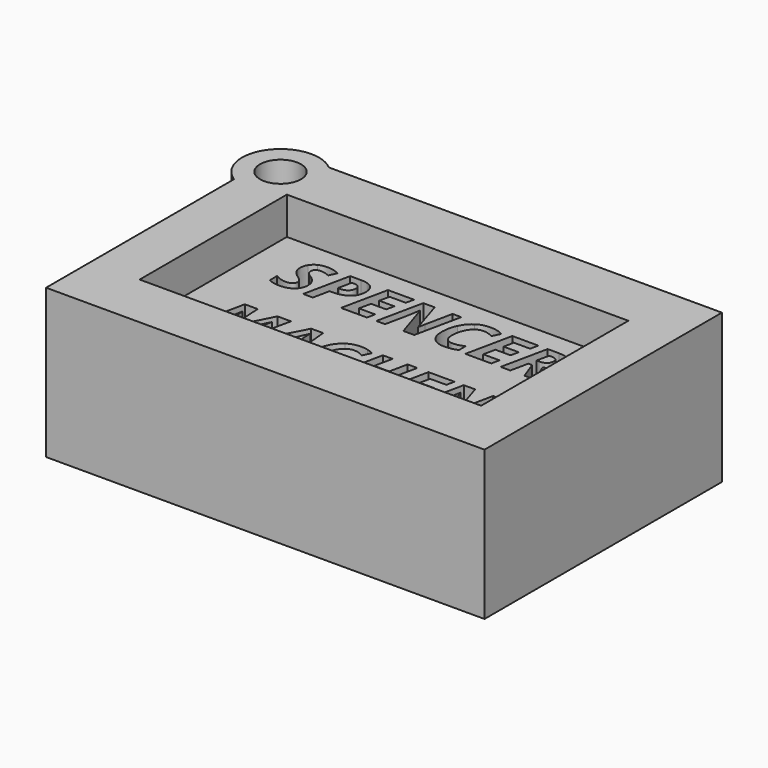
from build123d import *

# Parameters (mm, degrees)
F0_W         = 58.1890940666
F0_H         = 31.3483476639
F1_DEPTH     = 6.35
F2_DEPTH     = 25.4
F3_DEPTH     = 12.7
F4_DEPTH     = 12.7
F0_TEXT_SIZE = 11.0982710289
F5_DEPTH     = 12.7
F6_DEPTH     = 19.05


# Not quite as in the source:
# - Text() gives the source's letters only with a copy of the font that has no kerning and outlines rounded to 1/6400 em; it was checked with that copy


with BuildPart() as f1:
    # F0 (on Top) → F1 (new body)
    with BuildSketch(Plane.XY):
        with BuildLine():
            Line((-37.3486888398, -25.2818514363), (37.3486888398, -25.2818514363))
            Line((37.3486888398, -25.2818514363), (37.3486888398, 25.2818514363))
            Line((37.3486888398, 25.2818514363), (-29.6175755934, 25.2818514363))
            ThreePointArc((-29.6175755934, 25.2818514363), (-27.9167987863, 23.0401985803), (-27.3127590842, 20.2919654548))
            ThreePointArc((-27.3127590842, 20.2919654548), (-30.6939014972, 14.5572193058), (-37.3486888398, 14.7395454853))
            Line((-37.3486888398, 14.7395454853), (-37.3486888398, -25.2818514363))
        make_face()
        Rectangle(F0_W, F0_H, mode=Mode.SUBTRACT)
        Rectangle(F0_W, F0_H)
        with BuildLine():
            Line((-18.7833381513, -8.8915199012), (-18.7607947882, -8.8915199012))
            Line((-18.7607947882, -8.8915199012), (-15.7746662395, -2.9678177396))
            Line((-15.7746662395, -2.9678177396), (-13.4821796301, -2.9678177396))
            Line((-13.4821796301, -2.9678177396), (-15.1573249136, -10.8909427913))
            Line((-15.1573249136, -10.8909427913), (-16.6746666558, -10.8909427913))
            Line((-16.6746666558, -10.8909427913), (-15.8891171595, -7.1400740045))
            add(Edge.make_bspline(
                [(-15.8891171595, -7.1400740045), (-15.6012557547, -5.8030791665), (-15.3203307693, -4.7504775236)],
                knots=[0, 0, 0, 1, 1, 1], degree=2))
            Line((-15.3203307693, -4.7504775236), (-15.346342342, -4.7504775236))
            Line((-15.346342342, -4.7504775236), (-18.4313148671, -10.8909427913))
            Line((-18.4313148671, -10.8909427913), (-19.9538589239, -10.8909427913))
            Line((-19.9538589239, -10.8909427913), (-20.283338845, -4.7504775236))
            Line((-20.283338845, -4.7504775236), (-20.305882208, -4.7504775236))
            add(Edge.make_bspline(
                [(-20.305882208, -4.7504775236), (-20.3648417729, -5.2273563569), (-20.5113736326, -6.002501224)],
                knots=[0, 0, 0, 1, 1, 1], degree=2))
            add(Edge.make_bspline(
                [(-20.5113736326, -6.002501224), (-20.6579054922, -6.7776460912), (-21.5249579164, -10.8909427913)],
                knots=[0, 0, 0, 1, 1, 1], degree=2))
            Line((-21.5249579164, -10.8909427913), (-23.014553981, -10.8909427913))
            Line((-23.014553981, -10.8909427913), (-21.3411428025, -2.9678177396))
            Line((-21.3411428025, -2.9678177396), (-19.1509683791, -2.9678177396))
            Line((-19.1509683791, -2.9678177396), (-18.7833381513, -8.8915199012))
        make_face(mode=Mode.SUBTRACT)
        Polygon((-8.8451832659, -10.8909427913), (-8.9752411295, -9.0042367164), (-11.5382480952, -9.0042367164), (-12.4694623988, -10.8909427913), (-14.203567247, -10.8909427913), (-10.0538543451, -2.9348697475), (-8.0318880921, -2.9348697475), (-7.2359339667, -10.8909427913), align=None, mode=Mode.SUBTRACT)
        with BuildLine():
            add(Edge.make_bspline(
                [(-0.9211911618, -4.3446969891), (-1.2948907566, -4.242384803), (-1.6642550893, -4.242384803)],
                knots=[0, 0, 0, 1, 1, 1], degree=2))
            add(Edge.make_bspline(
                [(-1.6642550893, -4.242384803), (-2.3787062867, -4.242384803), (-2.9509608867, -4.6811133297)],
                knots=[0, 0, 0, 1, 1, 1], degree=2))
            add(Edge.make_bspline(
                [(-2.9509608867, -4.6811133297), (-3.5232154866, -5.1198418563), (-3.8700364562, -5.9730214416)],
                knots=[0, 0, 0, 1, 1, 1], degree=2))
            add(Edge.make_bspline(
                [(-3.8700364562, -5.9730214416), (-4.2168574259, -6.8262010269), (-4.2168574259, -7.8077043711)],
                knots=[0, 0, 0, 1, 1, 1], degree=2))
            add(Edge.make_bspline(
                [(-4.2168574259, -7.8077043711), (-4.2168574259, -8.7129071019), (-3.8457589884, -9.1516356285)],
                knots=[0, 0, 0, 1, 1, 1], degree=2))
            add(Edge.make_bspline(
                [(-3.8457589884, -9.1516356285), (-3.4746605508, -9.5903641551), (-2.661365377, -9.5903641551)],
                knots=[0, 0, 0, 1, 1, 1], degree=2))
            add(Edge.make_bspline(
                [(-2.661365377, -9.5903641551), (-1.8706135662, -9.5903641551), (-0.8301506572, -9.1724448866)],
                knots=[0, 0, 0, 1, 1, 1], degree=2))
            Line((-0.8301506572, -9.1724448866), (-0.8301506572, -10.5822721283))
            add(Edge.make_bspline(
                [(-0.8301506572, -10.5822721283), (-1.907029768, -11.0001913967), (-2.9977817176, -11.0001913967)],
                knots=[0, 0, 0, 1, 1, 1], degree=2))
            add(Edge.make_bspline(
                [(-2.9977817176, -11.0001913967), (-4.3729268622, -11.0001913967), (-5.1376671003, -10.1894973801)],
                knots=[0, 0, 0, 1, 1, 1], degree=2))
            add(Edge.make_bspline(
                [(-5.1376671003, -10.1894973801), (-5.9024073384, -9.3788033636), (-5.9024073384, -7.8944096135)],
                knots=[0, 0, 0, 1, 1, 1], degree=2))
            add(Edge.make_bspline(
                [(-5.9024073384, -7.8944096135), (-5.9024073384, -6.4741777428), (-5.3388232627, -5.2793795023)],
                knots=[0, 0, 0, 1, 1, 1], degree=2))
            add(Edge.make_bspline(
                [(-5.3388232627, -5.2793795023), (-4.775239187, -4.0845812618), (-3.8318861496, -3.4637717262)],
                knots=[0, 0, 0, 1, 1, 1], degree=2))
            add(Edge.make_bspline(
                [(-3.8318861496, -3.4637717262), (-2.8885331121, -2.8429621905), (-1.6642550893, -2.8429621905)],
                knots=[0, 0, 0, 1, 1, 1], degree=2))
            add(Edge.make_bspline(
                [(-1.6642550893, -2.8429621905), (-0.9862200936, -2.8429621905), (-0.4607863246, -2.9652165823)],
                knots=[0, 0, 0, 1, 1, 1], degree=2))
            add(Edge.make_bspline(
                [(-0.4607863246, -2.9652165823), (0.0646474445, -3.0874709741), (0.6663818268, -3.4117485807)],
                knots=[0, 0, 0, 1, 1, 1], degree=2))
            Line((0.6663818268, -3.4117485807), (0.0264971378, -4.7678185721))
            add(Edge.make_bspline(
                [(0.0264971378, -4.7678185721), (-0.547491567, -4.4470091751), (-0.9211911618, -4.3446969891)],
                knots=[0, 0, 0, 1, 1, 1], degree=2))
        make_face(mode=Mode.SUBTRACT)
        Polygon((8.0484661658, -2.9678177396), (6.3733208824, -10.8909427913), (4.7155166475, -10.8909427913), (5.4403724741, -7.4712880305), (2.8895042423, -7.4712880305), (2.1629143109, -10.8909427913), (0.5103123905, -10.8909427913), (2.183723569, -2.9678177396), (3.8432619088, -2.9678177396), (3.1860361713, -6.0735995228), (5.738638508, -6.0735995228), (6.3941301406, -2.9678177396), align=None, mode=Mode.SUBTRACT)
        Polygon((13.0010696125, -9.5036589127), (12.7080058931, -10.8909427913), (8.2808362155, -10.8909427913), (9.9542473941, -2.9678177396), (14.3883534911, -2.9678177396), (14.0952897717, -4.3446969891), (11.3207220145, -4.3446969891), (10.9565599964, -6.0840041519), (13.5421103251, -6.0840041519), (13.2438442912, -7.4608834014), (10.6600280673, -7.4608834014), (10.2265018553, -9.5036589127), align=None, mode=Mode.SUBTRACT)
        with BuildLine():
            Line((22.4415364064, -2.9678177396), (20.766391123, -10.8909427913))
            Line((20.766391123, -10.8909427913), (18.9126330402, -10.8909427913))
            Line((18.9126330402, -10.8909427913), (16.9843084489, -4.8978764357))
            Line((16.9843084489, -4.8978764357), (16.9513604568, -4.8978764357))
            Line((16.9513604568, -4.8978764357), (16.9288170938, -5.0712869205))
            add(Edge.make_bspline(
                [(16.9288170938, -5.0712869205), (16.755406609, -6.2418076931), (16.571591495, -7.1626173675)],
                knots=[0, 0, 0, 1, 1, 1], degree=2))
            Line((16.571591495, -7.1626173675), (15.7860419988, -10.8909427913))
            Line((15.7860419988, -10.8909427913), (14.2964459341, -10.8909427913))
            Line((14.2964459341, -10.8909427913), (15.9698571127, -2.9678177396))
            Line((15.9698571127, -2.9678177396), (17.9051181234, -2.9678177396))
            Line((17.9051181234, -2.9678177396), (19.7467374722, -8.8048146588))
            Line((19.7467374722, -8.8048146588), (19.7692808352, -8.8048146588))
            add(Edge.make_bspline(
                [(19.7692808352, -8.8048146588), (19.8334427146, -8.3920977049), (19.9799745743, -7.6282245193)],
                knots=[0, 0, 0, 1, 1, 1], degree=2))
            add(Edge.make_bspline(
                [(19.9799745743, -7.6282245193), (20.126506434, -6.8643513336), (20.9554085514, -2.9678177396)],
                knots=[0, 0, 0, 1, 1, 1], degree=2))
            Line((20.9554085514, -2.9678177396), (22.4415364064, -2.9678177396))
        make_face(mode=Mode.SUBTRACT)
        with BuildLine():
            add(Edge.make_bspline(
                [(-18.5015461134, 7.7654242187), (-18.1764014544, 7.242591607), (-18.1764014544, 6.5437473531)],
                knots=[0, 0, 0, 1, 1, 1], degree=2))
            add(Edge.make_bspline(
                [(-18.1764014544, 6.5437473531), (-18.1764014544, 5.4113768872), (-18.9784249467, 4.7524170449)],
                knots=[0, 0, 0, 1, 1, 1], degree=2))
            add(Edge.make_bspline(
                [(-18.9784249467, 4.7524170449), (-19.780448439, 4.0934572025), (-21.1503912692, 4.0934572025)],
                knots=[0, 0, 0, 1, 1, 1], degree=2))
            add(Edge.make_bspline(
                [(-21.1503912692, 4.0934572025), (-22.3486577193, 4.0934572025), (-23.0804499653, 4.5824747698)],
                knots=[0, 0, 0, 1, 1, 1], degree=2))
            Line((-23.0804499653, 4.5824747698), (-23.0804499653, 6.0668685199))
            add(Edge.make_bspline(
                [(-23.0804499653, 6.0668685199), (-22.0347847418, 5.482475186), (-21.1399866401, 5.482475186)],
                knots=[0, 0, 0, 1, 1, 1], degree=2))
            add(Edge.make_bspline(
                [(-21.1399866401, 5.482475186), (-20.5330499432, 5.482475186), (-20.1914312881, 5.7122440784)],
                knots=[0, 0, 0, 1, 1, 1], degree=2))
            add(Edge.make_bspline(
                [(-20.1914312881, 5.7122440784), (-19.849812633, 5.9420129708), (-19.849812633, 6.3425911907)],
                knots=[0, 0, 0, 1, 1, 1], degree=2))
            add(Edge.make_bspline(
                [(-19.849812633, 6.3425911907), (-19.849812633, 6.5766953453), (-19.923512089, 6.7527069873)],
                knots=[0, 0, 0, 1, 1, 1], degree=2))
            add(Edge.make_bspline(
                [(-19.923512089, 6.7527069873), (-19.9972115451, 6.9287186294), (-20.1324717232, 7.0804528037)],
                knots=[0, 0, 0, 1, 1, 1], degree=2))
            add(Edge.make_bspline(
                [(-20.1324717232, 7.0804528037), (-20.2677319014, 7.2321869779), (-20.8035702995, 7.6327651978)],
                knots=[0, 0, 0, 1, 1, 1], degree=2))
            add(Edge.make_bspline(
                [(-20.8035702995, 7.6327651978), (-21.5527035939, 8.1703377008), (-21.8561719424, 8.6957714698)],
                knots=[0, 0, 0, 1, 1, 1], degree=2))
            add(Edge.make_bspline(
                [(-21.8561719424, 8.6957714698), (-22.1596402908, 9.2212052388), (-22.1596402908, 9.8281419357)],
                knots=[0, 0, 0, 1, 1, 1], degree=2))
            add(Edge.make_bspline(
                [(-22.1596402908, 9.8281419357), (-22.1596402908, 10.5269861896), (-21.8232239503, 11.0766974265)],
                knots=[0, 0, 0, 1, 1, 1], degree=2))
            add(Edge.make_bspline(
                [(-21.8232239503, 11.0766974265), (-21.4868076097, 11.6264086634), (-20.865998074, 11.9324781691)],
                knots=[0, 0, 0, 1, 1, 1], degree=2))
            add(Edge.make_bspline(
                [(-20.865998074, 11.9324781691), (-20.2451885384, 12.2385476748), (-19.4388297839, 12.2385476748)],
                knots=[0, 0, 0, 1, 1, 1], degree=2))
            add(Edge.make_bspline(
                [(-19.4388297839, 12.2385476748), (-18.2631066968, 12.2385476748), (-17.2868056672, 11.7027092767)],
                knots=[0, 0, 0, 1, 1, 1], degree=2))
            Line((-17.2868056672, 11.7027092767), (-17.8781354205, 10.4402809472))
            add(Edge.make_bspline(
                [(-17.8781354205, 10.4402809472), (-18.7226444816, 10.8408591671), (-19.4388297839, 10.8408591671)],
                knots=[0, 0, 0, 1, 1, 1], degree=2))
            add(Edge.make_bspline(
                [(-19.4388297839, 10.8408591671), (-19.8879629396, 10.8408591671), (-20.174957292, 10.5972174359)],
                knots=[0, 0, 0, 1, 1, 1], degree=2))
            add(Edge.make_bspline(
                [(-20.174957292, 10.5972174359), (-20.4619516444, 10.3535757048), (-20.4619516444, 9.9529974848)],
                knots=[0, 0, 0, 1, 1, 1], degree=2))
            add(Edge.make_bspline(
                [(-20.4619516444, 9.9529974848), (-20.4619516444, 9.6217834588), (-20.283338845, 9.3755405703)],
                knots=[0, 0, 0, 1, 1, 1], degree=2))
            add(Edge.make_bspline(
                [(-20.283338845, 9.3755405703), (-20.1047260457, 9.1292976819), (-19.4821824051, 8.7217830425)],
                knots=[0, 0, 0, 1, 1, 1], degree=2))
            add(Edge.make_bspline(
                [(-19.4821824051, 8.7217830425), (-18.8266907725, 8.2882568305), (-18.5015461134, 7.7654242187)],
                knots=[0, 0, 0, 1, 1, 1], degree=2))
        make_face(mode=Mode.SUBTRACT)
        with BuildLine():
            add(Edge.make_bspline(
                [(-11.6448955434, 11.5483739452), (-10.9729299147, 10.9709170307), (-10.9729299147, 9.8177373066)],
                knots=[0, 0, 0, 1, 1, 1], degree=2))
            add(Edge.make_bspline(
                [(-10.9729299147, 9.8177373066), (-10.9729299147, 8.5102222511), (-11.8920054843, 7.7654242187)],
                knots=[0, 0, 0, 1, 1, 1], degree=2))
            add(Edge.make_bspline(
                [(-11.8920054843, 7.7654242187), (-12.8110810539, 7.0206261864), (-14.4255326676, 7.0206261864)],
                knots=[0, 0, 0, 1, 1, 1], degree=2))
            Line((-14.4255326676, 7.0206261864), (-14.8920068718, 7.0206261864))
            Line((-14.8920068718, 7.0206261864), (-15.4816025202, 4.202705808))
            Line((-15.4816025202, 4.202705808), (-17.1342044406, 4.202705808))
            Line((-17.1342044406, 4.202705808), (-15.460793262, 12.1258308597))
            Line((-15.460793262, 12.1258308597), (-13.6278444374, 12.1258308597))
            add(Edge.make_bspline(
                [(-13.6278444374, 12.1258308597), (-12.3168611721, 12.1258308597), (-11.6448955434, 11.5483739452)],
                knots=[0, 0, 0, 1, 1, 1], degree=2))
        make_face(mode=Mode.SUBTRACT)
        Polygon((-5.975239742, 5.5899896866), (-6.2683034614, 4.202705808), (-10.695473139, 4.202705808), (-9.0220619604, 12.1258308597), (-4.5879558634, 12.1258308597), (-4.8810195828, 10.7489516102), (-7.65558734, 10.7489516102), (-8.0197493581, 9.0096444474), (-5.4341990294, 9.0096444474), (-5.7324650633, 7.6327651978), (-8.3162812872, 7.6327651978), (-8.7498074992, 5.5899896866), align=None, mode=Mode.SUBTRACT)
        with BuildLine():
            Line((3.4652270519, 12.1258308597), (1.7900817685, 4.202705808))
            Line((1.7900817685, 4.202705808), (-0.0636763143, 4.202705808))
            Line((-0.0636763143, 4.202705808), (-1.9920009056, 10.1957721636))
            Line((-1.9920009056, 10.1957721636), (-2.0249488977, 10.1957721636))
            Line((-2.0249488977, 10.1957721636), (-2.0474922607, 10.0223616787))
            add(Edge.make_bspline(
                [(-2.0474922607, 10.0223616787), (-2.2209027455, 8.8518409062), (-2.4047178595, 7.9310312317)],
                knots=[0, 0, 0, 1, 1, 1], degree=2))
            Line((-2.4047178595, 7.9310312317), (-3.1902673557, 4.202705808))
            Line((-3.1902673557, 4.202705808), (-4.6798634204, 4.202705808))
            Line((-4.6798634204, 4.202705808), (-3.0064522418, 12.1258308597))
            Line((-3.0064522418, 12.1258308597), (-1.0711912312, 12.1258308597))
            Line((-1.0711912312, 12.1258308597), (0.7704281177, 6.2888339404))
            Line((0.7704281177, 6.2888339404), (0.7929714807, 6.2888339404))
            add(Edge.make_bspline(
                [(0.7929714807, 6.2888339404), (0.8571333601, 6.7015508943), (1.0036652198, 7.46542408)],
                knots=[0, 0, 0, 1, 1, 1], degree=2))
            add(Edge.make_bspline(
                [(1.0036652198, 7.46542408), (1.1501970795, 8.2292972656), (1.9790991969, 12.1258308597)],
                knots=[0, 0, 0, 1, 1, 1], degree=2))
            Line((1.9790991969, 12.1258308597), (3.4652270519, 12.1258308597))
        make_face(mode=Mode.SUBTRACT)
        with BuildLine():
            add(Edge.make_bspline(
                [(9.0568481351, 10.7489516102), (8.6831485403, 10.8512637962), (8.3137842076, 10.8512637962)],
                knots=[0, 0, 0, 1, 1, 1], degree=2))
            add(Edge.make_bspline(
                [(8.3137842076, 10.8512637962), (7.5993330101, 10.8512637962), (7.0270784102, 10.4125352696)],
                knots=[0, 0, 0, 1, 1, 1], degree=2))
            add(Edge.make_bspline(
                [(7.0270784102, 10.4125352696), (6.4548238103, 9.973806743), (6.1080028406, 9.1206271576)],
                knots=[0, 0, 0, 1, 1, 1], degree=2))
            add(Edge.make_bspline(
                [(6.1080028406, 9.1206271576), (5.761181871, 8.2674475723), (5.761181871, 7.2859442282)],
                knots=[0, 0, 0, 1, 1, 1], degree=2))
            add(Edge.make_bspline(
                [(5.761181871, 7.2859442282), (5.761181871, 6.3807414974), (6.1322803085, 5.9420129708)],
                knots=[0, 0, 0, 1, 1, 1], degree=2))
            add(Edge.make_bspline(
                [(6.1322803085, 5.9420129708), (6.503378746, 5.5032844442), (7.3166739199, 5.5032844442)],
                knots=[0, 0, 0, 1, 1, 1], degree=2))
            add(Edge.make_bspline(
                [(7.3166739199, 5.5032844442), (8.1074257307, 5.5032844442), (9.1478886396, 5.9212037126)],
                knots=[0, 0, 0, 1, 1, 1], degree=2))
            Line((9.1478886396, 5.9212037126), (9.1478886396, 4.511376471))
            add(Edge.make_bspline(
                [(9.1478886396, 4.511376471), (8.0710095289, 4.0934572025), (6.9802575793, 4.0934572025)],
                knots=[0, 0, 0, 1, 1, 1], degree=2))
            add(Edge.make_bspline(
                [(6.9802575793, 4.0934572025), (5.6051124346, 4.0934572025), (4.8403721966, 4.9041512191)],
                knots=[0, 0, 0, 1, 1, 1], degree=2))
            add(Edge.make_bspline(
                [(4.8403721966, 4.9041512191), (4.0756319585, 5.7148452357), (4.0756319585, 7.1992389858)],
                knots=[0, 0, 0, 1, 1, 1], degree=2))
            add(Edge.make_bspline(
                [(4.0756319585, 7.1992389858), (4.0756319585, 8.6194708565), (4.6392160342, 9.814269097)],
                knots=[0, 0, 0, 1, 1, 1], degree=2))
            add(Edge.make_bspline(
                [(4.6392160342, 9.814269097), (5.2028001099, 11.0090673374), (6.1461531473, 11.6298768731)],
                knots=[0, 0, 0, 1, 1, 1], degree=2))
            add(Edge.make_bspline(
                [(6.1461531473, 11.6298768731), (7.0895061848, 12.2506864088), (8.3137842076, 12.2506864088)],
                knots=[0, 0, 0, 1, 1, 1], degree=2))
            add(Edge.make_bspline(
                [(8.3137842076, 12.2506864088), (8.9918192033, 12.2506864088), (9.5172529723, 12.128432017)],
                knots=[0, 0, 0, 1, 1, 1], degree=2))
            add(Edge.make_bspline(
                [(9.5172529723, 12.128432017), (10.0426867413, 12.0061776252), (10.6444211237, 11.6819000185)],
                knots=[0, 0, 0, 1, 1, 1], degree=2))
            Line((10.6444211237, 11.6819000185), (10.0045364347, 10.3258300272))
            add(Edge.make_bspline(
                [(10.0045364347, 10.3258300272), (9.4305477299, 10.6466394241), (9.0568481351, 10.7489516102)],
                knots=[0, 0, 0, 1, 1, 1], degree=2))
        make_face(mode=Mode.SUBTRACT)
        Polygon((15.2085850843, 5.5899896866), (14.915521365, 4.202705808), (10.4883516873, 4.202705808), (12.1617628659, 12.1258308597), (16.5958689629, 12.1258308597), (16.3028052436, 10.7489516102), (13.5282374863, 10.7489516102), (13.1640754682, 9.0096444474), (15.749625797, 9.0096444474), (15.4513597631, 7.6327651978), (12.8675435392, 7.6327651978), (12.4340173271, 5.5899896866), align=None, mode=Mode.SUBTRACT)
        with BuildLine():
            Line((19.4467373335, 7.242591607), (18.8016503299, 7.242591607))
            Line((18.8016503299, 7.242591607), (18.1565633264, 4.202705808))
            Line((18.1565633264, 4.202705808), (16.503961406, 4.202705808))
            Line((16.503961406, 4.202705808), (18.1773725845, 12.1258308597))
            Line((18.1773725845, 12.1258308597), (20.1230382243, 12.1258308597))
            add(Edge.make_bspline(
                [(20.1230382243, 12.1258308597), (21.4080099168, 12.1258308597), (22.0530969204, 11.5726514131)],
                knots=[0, 0, 0, 1, 1, 1], degree=2))
            add(Edge.make_bspline(
                [(22.0530969204, 11.5726514131), (22.6981839239, 11.0194719665), (22.6981839239, 9.9529974848)],
                knots=[0, 0, 0, 1, 1, 1], degree=2))
            add(Edge.make_bspline(
                [(22.6981839239, 9.9529974848), (22.6981839239, 9.0963496898), (22.2481837158, 8.4816095211)],
                knots=[0, 0, 0, 1, 1, 1], degree=2))
            add(Edge.make_bspline(
                [(22.2481837158, 8.4816095211), (21.7981835077, 7.8668693524), (20.9519403417, 7.5686033185)],
                knots=[0, 0, 0, 1, 1, 1], degree=2))
            Line((20.9519403417, 7.5686033185), (22.3669698979, 4.202705808))
            Line((22.3669698979, 4.202705808), (20.5669690654, 4.202705808))
            Line((20.5669690654, 4.202705808), (19.4467373335, 7.242591607))
        make_face(mode=Mode.SUBTRACT)
        with BuildLine():
            Line((-0.0636763143, 4.202705808), (1.7900817685, 4.202705808))
            Line((1.7900817685, 4.202705808), (3.4652270519, 12.1258308597))
            Line((3.4652270519, 12.1258308597), (1.9790991969, 12.1258308597))
            add(Edge.make_bspline(
                [(1.0036652198, 7.46542408), (1.1501970795, 8.2292972656), (1.9790991969, 12.1258308597)],
                knots=[0, 0, 0, 1, 1, 1], degree=2))
            add(Edge.make_bspline(
                [(0.7929714807, 6.2888339404), (0.8571333601, 6.7015508943), (1.0036652198, 7.46542408)],
                knots=[0, 0, 0, 1, 1, 1], degree=2))
            Line((0.7929714807, 6.2888339404), (0.7704281177, 6.2888339404))
            Line((0.7704281177, 6.2888339404), (-1.0711912312, 12.1258308597))
            Line((-1.0711912312, 12.1258308597), (-3.0064522418, 12.1258308597))
            Line((-3.0064522418, 12.1258308597), (-4.6798634204, 4.202705808))
            Line((-4.6798634204, 4.202705808), (-3.1902673557, 4.202705808))
            Line((-3.1902673557, 4.202705808), (-2.4047178595, 7.9310312317))
            add(Edge.make_bspline(
                [(-2.0474922607, 10.0223616787), (-2.2209027455, 8.8518409062), (-2.4047178595, 7.9310312317)],
                knots=[0, 0, 0, 1, 1, 1], degree=2))
            Line((-2.0474922607, 10.0223616787), (-2.0249488977, 10.1957721636))
            Line((-2.0249488977, 10.1957721636), (-1.9920009056, 10.1957721636))
            Line((-1.9920009056, 10.1957721636), (-0.0636763143, 4.202705808))
        make_face()
        with BuildLine():
            add(Edge.make_bspline(
                [(8.3137842076, 10.8512637962), (7.5993330101, 10.8512637962), (7.0270784102, 10.4125352696)],
                knots=[0, 0, 0, 1, 1, 1], degree=2))
            add(Edge.make_bspline(
                [(9.0568481351, 10.7489516102), (8.6831485403, 10.8512637962), (8.3137842076, 10.8512637962)],
                knots=[0, 0, 0, 1, 1, 1], degree=2))
            add(Edge.make_bspline(
                [(10.0045364347, 10.3258300272), (9.4305477299, 10.6466394241), (9.0568481351, 10.7489516102)],
                knots=[0, 0, 0, 1, 1, 1], degree=2))
            Line((10.0045364347, 10.3258300272), (10.6444211237, 11.6819000185))
            add(Edge.make_bspline(
                [(9.5172529723, 12.128432017), (10.0426867413, 12.0061776252), (10.6444211237, 11.6819000185)],
                knots=[0, 0, 0, 1, 1, 1], degree=2))
            add(Edge.make_bspline(
                [(8.3137842076, 12.2506864088), (8.9918192033, 12.2506864088), (9.5172529723, 12.128432017)],
                knots=[0, 0, 0, 1, 1, 1], degree=2))
            add(Edge.make_bspline(
                [(6.1461531473, 11.6298768731), (7.0895061848, 12.2506864088), (8.3137842076, 12.2506864088)],
                knots=[0, 0, 0, 1, 1, 1], degree=2))
            add(Edge.make_bspline(
                [(4.6392160342, 9.814269097), (5.2028001099, 11.0090673374), (6.1461531473, 11.6298768731)],
                knots=[0, 0, 0, 1, 1, 1], degree=2))
            add(Edge.make_bspline(
                [(4.0756319585, 7.1992389858), (4.0756319585, 8.6194708565), (4.6392160342, 9.814269097)],
                knots=[0, 0, 0, 1, 1, 1], degree=2))
            add(Edge.make_bspline(
                [(4.8403721966, 4.9041512191), (4.0756319585, 5.7148452357), (4.0756319585, 7.1992389858)],
                knots=[0, 0, 0, 1, 1, 1], degree=2))
            add(Edge.make_bspline(
                [(6.9802575793, 4.0934572025), (5.6051124346, 4.0934572025), (4.8403721966, 4.9041512191)],
                knots=[0, 0, 0, 1, 1, 1], degree=2))
            add(Edge.make_bspline(
                [(9.1478886396, 4.511376471), (8.0710095289, 4.0934572025), (6.9802575793, 4.0934572025)],
                knots=[0, 0, 0, 1, 1, 1], degree=2))
            Line((9.1478886396, 4.511376471), (9.1478886396, 5.9212037126))
            add(Edge.make_bspline(
                [(7.3166739199, 5.5032844442), (8.1074257307, 5.5032844442), (9.1478886396, 5.9212037126)],
                knots=[0, 0, 0, 1, 1, 1], degree=2))
            add(Edge.make_bspline(
                [(6.1322803085, 5.9420129708), (6.503378746, 5.5032844442), (7.3166739199, 5.5032844442)],
                knots=[0, 0, 0, 1, 1, 1], degree=2))
            add(Edge.make_bspline(
                [(5.761181871, 7.2859442282), (5.761181871, 6.3807414974), (6.1322803085, 5.9420129708)],
                knots=[0, 0, 0, 1, 1, 1], degree=2))
            add(Edge.make_bspline(
                [(6.1080028406, 9.1206271576), (5.761181871, 8.2674475723), (5.761181871, 7.2859442282)],
                knots=[0, 0, 0, 1, 1, 1], degree=2))
            add(Edge.make_bspline(
                [(7.0270784102, 10.4125352696), (6.4548238103, 9.973806743), (6.1080028406, 9.1206271576)],
                knots=[0, 0, 0, 1, 1, 1], degree=2))
        make_face()
        with BuildLine():
            add(Edge.make_bspline(
                [(-18.1764014544, 6.5437473531), (-18.1764014544, 5.4113768872), (-18.9784249467, 4.7524170449)],
                knots=[0, 0, 0, 1, 1, 1], degree=2))
            add(Edge.make_bspline(
                [(-18.5015461134, 7.7654242187), (-18.1764014544, 7.242591607), (-18.1764014544, 6.5437473531)],
                knots=[0, 0, 0, 1, 1, 1], degree=2))
            add(Edge.make_bspline(
                [(-19.4821824051, 8.7217830425), (-18.8266907725, 8.2882568305), (-18.5015461134, 7.7654242187)],
                knots=[0, 0, 0, 1, 1, 1], degree=2))
            add(Edge.make_bspline(
                [(-20.283338845, 9.3755405703), (-20.1047260457, 9.1292976819), (-19.4821824051, 8.7217830425)],
                knots=[0, 0, 0, 1, 1, 1], degree=2))
            add(Edge.make_bspline(
                [(-20.4619516444, 9.9529974848), (-20.4619516444, 9.6217834588), (-20.283338845, 9.3755405703)],
                knots=[0, 0, 0, 1, 1, 1], degree=2))
            add(Edge.make_bspline(
                [(-20.174957292, 10.5972174359), (-20.4619516444, 10.3535757048), (-20.4619516444, 9.9529974848)],
                knots=[0, 0, 0, 1, 1, 1], degree=2))
            add(Edge.make_bspline(
                [(-19.4388297839, 10.8408591671), (-19.8879629396, 10.8408591671), (-20.174957292, 10.5972174359)],
                knots=[0, 0, 0, 1, 1, 1], degree=2))
            add(Edge.make_bspline(
                [(-17.8781354205, 10.4402809472), (-18.7226444816, 10.8408591671), (-19.4388297839, 10.8408591671)],
                knots=[0, 0, 0, 1, 1, 1], degree=2))
            Line((-17.8781354205, 10.4402809472), (-17.2868056672, 11.7027092767))
            add(Edge.make_bspline(
                [(-19.4388297839, 12.2385476748), (-18.2631066968, 12.2385476748), (-17.2868056672, 11.7027092767)],
                knots=[0, 0, 0, 1, 1, 1], degree=2))
            add(Edge.make_bspline(
                [(-20.865998074, 11.9324781691), (-20.2451885384, 12.2385476748), (-19.4388297839, 12.2385476748)],
                knots=[0, 0, 0, 1, 1, 1], degree=2))
            add(Edge.make_bspline(
                [(-21.8232239503, 11.0766974265), (-21.4868076097, 11.6264086634), (-20.865998074, 11.9324781691)],
                knots=[0, 0, 0, 1, 1, 1], degree=2))
            add(Edge.make_bspline(
                [(-22.1596402908, 9.8281419357), (-22.1596402908, 10.5269861896), (-21.8232239503, 11.0766974265)],
                knots=[0, 0, 0, 1, 1, 1], degree=2))
            add(Edge.make_bspline(
                [(-21.8561719424, 8.6957714698), (-22.1596402908, 9.2212052388), (-22.1596402908, 9.8281419357)],
                knots=[0, 0, 0, 1, 1, 1], degree=2))
            add(Edge.make_bspline(
                [(-20.8035702995, 7.6327651978), (-21.5527035939, 8.1703377008), (-21.8561719424, 8.6957714698)],
                knots=[0, 0, 0, 1, 1, 1], degree=2))
            add(Edge.make_bspline(
                [(-20.1324717232, 7.0804528037), (-20.2677319014, 7.2321869779), (-20.8035702995, 7.6327651978)],
                knots=[0, 0, 0, 1, 1, 1], degree=2))
            add(Edge.make_bspline(
                [(-19.923512089, 6.7527069873), (-19.9972115451, 6.9287186294), (-20.1324717232, 7.0804528037)],
                knots=[0, 0, 0, 1, 1, 1], degree=2))
            add(Edge.make_bspline(
                [(-19.849812633, 6.3425911907), (-19.849812633, 6.5766953453), (-19.923512089, 6.7527069873)],
                knots=[0, 0, 0, 1, 1, 1], degree=2))
            add(Edge.make_bspline(
                [(-20.1914312881, 5.7122440784), (-19.849812633, 5.9420129708), (-19.849812633, 6.3425911907)],
                knots=[0, 0, 0, 1, 1, 1], degree=2))
            add(Edge.make_bspline(
                [(-21.1399866401, 5.482475186), (-20.5330499432, 5.482475186), (-20.1914312881, 5.7122440784)],
                knots=[0, 0, 0, 1, 1, 1], degree=2))
            add(Edge.make_bspline(
                [(-23.0804499653, 6.0668685199), (-22.0347847418, 5.482475186), (-21.1399866401, 5.482475186)],
                knots=[0, 0, 0, 1, 1, 1], degree=2))
            Line((-23.0804499653, 6.0668685199), (-23.0804499653, 4.5824747698))
            add(Edge.make_bspline(
                [(-21.1503912692, 4.0934572025), (-22.3486577193, 4.0934572025), (-23.0804499653, 4.5824747698)],
                knots=[0, 0, 0, 1, 1, 1], degree=2))
            add(Edge.make_bspline(
                [(-18.9784249467, 4.7524170449), (-19.780448439, 4.0934572025), (-21.1503912692, 4.0934572025)],
                knots=[0, 0, 0, 1, 1, 1], degree=2))
        make_face()
        Polygon((-10.695473139, 4.202705808), (-6.2683034614, 4.202705808), (-5.975239742, 5.5899896866), (-8.7498074992, 5.5899896866), (-8.3162812872, 7.6327651978), (-5.7324650633, 7.6327651978), (-5.4341990294, 9.0096444474), (-8.0197493581, 9.0096444474), (-7.65558734, 10.7489516102), (-4.8810195828, 10.7489516102), (-4.5879558634, 12.1258308597), (-9.0220619604, 12.1258308597), align=None)
    extrude(amount=F1_DEPTH)

    # F0 (on Top) → F2 (join)
    with BuildSketch(Plane.XY):
        with BuildLine():
            Line((-37.3486888398, -25.2818514363), (37.3486888398, -25.2818514363))
            Line((37.3486888398, -25.2818514363), (37.3486888398, 25.2818514363))
            Line((37.3486888398, 25.2818514363), (-29.6175755934, 25.2818514363))
            ThreePointArc((-29.6175755934, 25.2818514363), (-27.9167987863, 23.0401985803), (-27.3127590842, 20.2919654548))
            ThreePointArc((-27.3127590842, 20.2919654548), (-30.6939014972, 14.5572193058), (-37.3486888398, 14.7395454853))
            Line((-37.3486888398, 14.7395454853), (-37.3486888398, -25.2818514363))
        make_face()
        Rectangle(F0_W, F0_H, mode=Mode.SUBTRACT)
        with BuildLine():
            ThreePointArc((-29.6175755934, 25.2818514363), (-39.1517619538, 24.1677413938), (-37.3486888398, 14.7395454853))
            Line((-37.3486888398, 14.7395454853), (-37.3486888398, 20.2919654548))
            Line((-37.3486888398, 20.2919654548), (-37.3486888398, 25.2818514363))
            Line((-37.3486888398, 25.2818514363), (-29.6175755934, 25.2818514363))
        make_face()
        with BuildLine():
            Line((-37.3486888398, 20.2919654548), (-37.3486888398, 14.7395454853))
            ThreePointArc((-37.3486888398, 14.7395454853), (-30.6939014972, 14.5572193058), (-27.3127590842, 20.2919654548))
            ThreePointArc((-27.3127590842, 20.2919654548), (-27.9167987863, 23.0401985803), (-29.6175755934, 25.2818514363))
            Line((-29.6175755934, 25.2818514363), (-37.3486888398, 25.2818514363))
            Line((-37.3486888398, 25.2818514363), (-37.3486888398, 20.2919654548))
        make_face()
        with BuildLine():
            ThreePointArc((-30.3846585762, 20.2919654548), (-33.866673708, 16.809950323), (-37.3486888398, 20.2919654548))
            ThreePointArc((-37.3486888398, 20.2919654548), (-33.866673708, 23.7739805866), (-30.3846585762, 20.2919654548))
        make_face(mode=Mode.SUBTRACT)
    extrude(amount=F2_DEPTH)

    # F0 (on Top) → F3 (join)
    with BuildSketch(Plane.XY):
        with BuildLine():
            add(Edge.make_bspline(
                [(-18.1764014544, 6.5437473531), (-18.1764014544, 5.4113768872), (-18.9784249467, 4.7524170449)],
                knots=[0, 0, 0, 1, 1, 1], degree=2))
            add(Edge.make_bspline(
                [(-18.5015461134, 7.7654242187), (-18.1764014544, 7.242591607), (-18.1764014544, 6.5437473531)],
                knots=[0, 0, 0, 1, 1, 1], degree=2))
            add(Edge.make_bspline(
                [(-19.4821824051, 8.7217830425), (-18.8266907725, 8.2882568305), (-18.5015461134, 7.7654242187)],
                knots=[0, 0, 0, 1, 1, 1], degree=2))
            add(Edge.make_bspline(
                [(-20.283338845, 9.3755405703), (-20.1047260457, 9.1292976819), (-19.4821824051, 8.7217830425)],
                knots=[0, 0, 0, 1, 1, 1], degree=2))
            add(Edge.make_bspline(
                [(-20.4619516444, 9.9529974848), (-20.4619516444, 9.6217834588), (-20.283338845, 9.3755405703)],
                knots=[0, 0, 0, 1, 1, 1], degree=2))
            add(Edge.make_bspline(
                [(-20.174957292, 10.5972174359), (-20.4619516444, 10.3535757048), (-20.4619516444, 9.9529974848)],
                knots=[0, 0, 0, 1, 1, 1], degree=2))
            add(Edge.make_bspline(
                [(-19.4388297839, 10.8408591671), (-19.8879629396, 10.8408591671), (-20.174957292, 10.5972174359)],
                knots=[0, 0, 0, 1, 1, 1], degree=2))
            add(Edge.make_bspline(
                [(-17.8781354205, 10.4402809472), (-18.7226444816, 10.8408591671), (-19.4388297839, 10.8408591671)],
                knots=[0, 0, 0, 1, 1, 1], degree=2))
            Line((-17.8781354205, 10.4402809472), (-17.2868056672, 11.7027092767))
            add(Edge.make_bspline(
                [(-19.4388297839, 12.2385476748), (-18.2631066968, 12.2385476748), (-17.2868056672, 11.7027092767)],
                knots=[0, 0, 0, 1, 1, 1], degree=2))
            add(Edge.make_bspline(
                [(-20.865998074, 11.9324781691), (-20.2451885384, 12.2385476748), (-19.4388297839, 12.2385476748)],
                knots=[0, 0, 0, 1, 1, 1], degree=2))
            add(Edge.make_bspline(
                [(-21.8232239503, 11.0766974265), (-21.4868076097, 11.6264086634), (-20.865998074, 11.9324781691)],
                knots=[0, 0, 0, 1, 1, 1], degree=2))
            add(Edge.make_bspline(
                [(-22.1596402908, 9.8281419357), (-22.1596402908, 10.5269861896), (-21.8232239503, 11.0766974265)],
                knots=[0, 0, 0, 1, 1, 1], degree=2))
            add(Edge.make_bspline(
                [(-21.8561719424, 8.6957714698), (-22.1596402908, 9.2212052388), (-22.1596402908, 9.8281419357)],
                knots=[0, 0, 0, 1, 1, 1], degree=2))
            add(Edge.make_bspline(
                [(-20.8035702995, 7.6327651978), (-21.5527035939, 8.1703377008), (-21.8561719424, 8.6957714698)],
                knots=[0, 0, 0, 1, 1, 1], degree=2))
            add(Edge.make_bspline(
                [(-20.1324717232, 7.0804528037), (-20.2677319014, 7.2321869779), (-20.8035702995, 7.6327651978)],
                knots=[0, 0, 0, 1, 1, 1], degree=2))
            add(Edge.make_bspline(
                [(-19.923512089, 6.7527069873), (-19.9972115451, 6.9287186294), (-20.1324717232, 7.0804528037)],
                knots=[0, 0, 0, 1, 1, 1], degree=2))
            add(Edge.make_bspline(
                [(-19.849812633, 6.3425911907), (-19.849812633, 6.5766953453), (-19.923512089, 6.7527069873)],
                knots=[0, 0, 0, 1, 1, 1], degree=2))
            add(Edge.make_bspline(
                [(-20.1914312881, 5.7122440784), (-19.849812633, 5.9420129708), (-19.849812633, 6.3425911907)],
                knots=[0, 0, 0, 1, 1, 1], degree=2))
            add(Edge.make_bspline(
                [(-21.1399866401, 5.482475186), (-20.5330499432, 5.482475186), (-20.1914312881, 5.7122440784)],
                knots=[0, 0, 0, 1, 1, 1], degree=2))
            add(Edge.make_bspline(
                [(-23.0804499653, 6.0668685199), (-22.0347847418, 5.482475186), (-21.1399866401, 5.482475186)],
                knots=[0, 0, 0, 1, 1, 1], degree=2))
            Line((-23.0804499653, 6.0668685199), (-23.0804499653, 4.5824747698))
            add(Edge.make_bspline(
                [(-21.1503912692, 4.0934572025), (-22.3486577193, 4.0934572025), (-23.0804499653, 4.5824747698)],
                knots=[0, 0, 0, 1, 1, 1], degree=2))
            add(Edge.make_bspline(
                [(-18.9784249467, 4.7524170449), (-19.780448439, 4.0934572025), (-21.1503912692, 4.0934572025)],
                knots=[0, 0, 0, 1, 1, 1], degree=2))
        make_face()
        Polygon((-10.695473139, 4.202705808), (-6.2683034614, 4.202705808), (-5.975239742, 5.5899896866), (-8.7498074992, 5.5899896866), (-8.3162812872, 7.6327651978), (-5.7324650633, 7.6327651978), (-5.4341990294, 9.0096444474), (-8.0197493581, 9.0096444474), (-7.65558734, 10.7489516102), (-4.8810195828, 10.7489516102), (-4.5879558634, 12.1258308597), (-9.0220619604, 12.1258308597), align=None)
        with BuildLine():
            Line((-0.0636763143, 4.202705808), (1.7900817685, 4.202705808))
            Line((1.7900817685, 4.202705808), (3.4652270519, 12.1258308597))
            Line((3.4652270519, 12.1258308597), (1.9790991969, 12.1258308597))
            add(Edge.make_bspline(
                [(1.0036652198, 7.46542408), (1.1501970795, 8.2292972656), (1.9790991969, 12.1258308597)],
                knots=[0, 0, 0, 1, 1, 1], degree=2))
            add(Edge.make_bspline(
                [(0.7929714807, 6.2888339404), (0.8571333601, 6.7015508943), (1.0036652198, 7.46542408)],
                knots=[0, 0, 0, 1, 1, 1], degree=2))
            Line((0.7929714807, 6.2888339404), (0.7704281177, 6.2888339404))
            Line((0.7704281177, 6.2888339404), (-1.0711912312, 12.1258308597))
            Line((-1.0711912312, 12.1258308597), (-3.0064522418, 12.1258308597))
            Line((-3.0064522418, 12.1258308597), (-4.6798634204, 4.202705808))
            Line((-4.6798634204, 4.202705808), (-3.1902673557, 4.202705808))
            Line((-3.1902673557, 4.202705808), (-2.4047178595, 7.9310312317))
            add(Edge.make_bspline(
                [(-2.0474922607, 10.0223616787), (-2.2209027455, 8.8518409062), (-2.4047178595, 7.9310312317)],
                knots=[0, 0, 0, 1, 1, 1], degree=2))
            Line((-2.0474922607, 10.0223616787), (-2.0249488977, 10.1957721636))
            Line((-2.0249488977, 10.1957721636), (-1.9920009056, 10.1957721636))
            Line((-1.9920009056, 10.1957721636), (-0.0636763143, 4.202705808))
        make_face()
        with BuildLine():
            add(Edge.make_bspline(
                [(8.3137842076, 10.8512637962), (7.5993330101, 10.8512637962), (7.0270784102, 10.4125352696)],
                knots=[0, 0, 0, 1, 1, 1], degree=2))
            add(Edge.make_bspline(
                [(9.0568481351, 10.7489516102), (8.6831485403, 10.8512637962), (8.3137842076, 10.8512637962)],
                knots=[0, 0, 0, 1, 1, 1], degree=2))
            add(Edge.make_bspline(
                [(10.0045364347, 10.3258300272), (9.4305477299, 10.6466394241), (9.0568481351, 10.7489516102)],
                knots=[0, 0, 0, 1, 1, 1], degree=2))
            Line((10.0045364347, 10.3258300272), (10.6444211237, 11.6819000185))
            add(Edge.make_bspline(
                [(9.5172529723, 12.128432017), (10.0426867413, 12.0061776252), (10.6444211237, 11.6819000185)],
                knots=[0, 0, 0, 1, 1, 1], degree=2))
            add(Edge.make_bspline(
                [(8.3137842076, 12.2506864088), (8.9918192033, 12.2506864088), (9.5172529723, 12.128432017)],
                knots=[0, 0, 0, 1, 1, 1], degree=2))
            add(Edge.make_bspline(
                [(6.1461531473, 11.6298768731), (7.0895061848, 12.2506864088), (8.3137842076, 12.2506864088)],
                knots=[0, 0, 0, 1, 1, 1], degree=2))
            add(Edge.make_bspline(
                [(4.6392160342, 9.814269097), (5.2028001099, 11.0090673374), (6.1461531473, 11.6298768731)],
                knots=[0, 0, 0, 1, 1, 1], degree=2))
            add(Edge.make_bspline(
                [(4.0756319585, 7.1992389858), (4.0756319585, 8.6194708565), (4.6392160342, 9.814269097)],
                knots=[0, 0, 0, 1, 1, 1], degree=2))
            add(Edge.make_bspline(
                [(4.8403721966, 4.9041512191), (4.0756319585, 5.7148452357), (4.0756319585, 7.1992389858)],
                knots=[0, 0, 0, 1, 1, 1], degree=2))
            add(Edge.make_bspline(
                [(6.9802575793, 4.0934572025), (5.6051124346, 4.0934572025), (4.8403721966, 4.9041512191)],
                knots=[0, 0, 0, 1, 1, 1], degree=2))
            add(Edge.make_bspline(
                [(9.1478886396, 4.511376471), (8.0710095289, 4.0934572025), (6.9802575793, 4.0934572025)],
                knots=[0, 0, 0, 1, 1, 1], degree=2))
            Line((9.1478886396, 4.511376471), (9.1478886396, 5.9212037126))
            add(Edge.make_bspline(
                [(7.3166739199, 5.5032844442), (8.1074257307, 5.5032844442), (9.1478886396, 5.9212037126)],
                knots=[0, 0, 0, 1, 1, 1], degree=2))
            add(Edge.make_bspline(
                [(6.1322803085, 5.9420129708), (6.503378746, 5.5032844442), (7.3166739199, 5.5032844442)],
                knots=[0, 0, 0, 1, 1, 1], degree=2))
            add(Edge.make_bspline(
                [(5.761181871, 7.2859442282), (5.761181871, 6.3807414974), (6.1322803085, 5.9420129708)],
                knots=[0, 0, 0, 1, 1, 1], degree=2))
            add(Edge.make_bspline(
                [(6.1080028406, 9.1206271576), (5.761181871, 8.2674475723), (5.761181871, 7.2859442282)],
                knots=[0, 0, 0, 1, 1, 1], degree=2))
            add(Edge.make_bspline(
                [(7.0270784102, 10.4125352696), (6.4548238103, 9.973806743), (6.1080028406, 9.1206271576)],
                knots=[0, 0, 0, 1, 1, 1], degree=2))
        make_face()
    extrude(amount=F3_DEPTH)

    # F4 (add): a face of the model
    f4_faces = [f1.faces().sort_by_distance(p)[0] for p in [
        (0.0651923339, -0.2017890661, 6.35),
    ]]
    extrude(f4_faces, amount=F4_DEPTH)

    # F0 (on Top) → F5 (join)
    with BuildSketch(Plane.XY):
        with BuildLine():
            add(Edge.make_bspline(
                [(-10.9729299147, 9.8177373066), (-10.9729299147, 8.5102222511), (-11.8920054843, 7.7654242187)],
                knots=[0, 0, 0, 1, 1, 1], degree=2))
            add(Edge.make_bspline(
                [(-11.6448955434, 11.5483739452), (-10.9729299147, 10.9709170307), (-10.9729299147, 9.8177373066)],
                knots=[0, 0, 0, 1, 1, 1], degree=2))
            add(Edge.make_bspline(
                [(-13.6278444374, 12.1258308597), (-12.3168611721, 12.1258308597), (-11.6448955434, 11.5483739452)],
                knots=[0, 0, 0, 1, 1, 1], degree=2))
            Line((-13.6278444374, 12.1258308597), (-15.460793262, 12.1258308597))
            Line((-15.460793262, 12.1258308597), (-17.1342044406, 4.202705808))
            Line((-17.1342044406, 4.202705808), (-15.4816025202, 4.202705808))
            Line((-15.4816025202, 4.202705808), (-14.8920068718, 7.0206261864))
            Line((-14.8920068718, 7.0206261864), (-14.4255326676, 7.0206261864))
            add(Edge.make_bspline(
                [(-11.8920054843, 7.7654242187), (-12.8110810539, 7.0206261864), (-14.4255326676, 7.0206261864)],
                knots=[0, 0, 0, 1, 1, 1], degree=2))
        make_face()
        with BuildLine():
            Line((-14.2902724894, 8.3975054359), (-14.5937408379, 8.3975054359))
            Line((-14.5937408379, 8.3975054359), (-14.0943186416, 10.7489516102))
            Line((-14.0943186416, 10.7489516102), (-13.6937404216, 10.7489516102))
            add(Edge.make_bspline(
                [(-12.637670569, 9.7743846854), (-12.637670569, 10.7489516102), (-13.6937404216, 10.7489516102)],
                knots=[0, 0, 0, 1, 1, 1], degree=2))
            add(Edge.make_bspline(
                [(-13.0790002529, 8.7712050307), (-12.637670569, 9.1449046255), (-12.637670569, 9.7743846854)],
                knots=[0, 0, 0, 1, 1, 1], degree=2))
            add(Edge.make_bspline(
                [(-14.2902724894, 8.3975054359), (-13.5203299368, 8.3975054359), (-13.0790002529, 8.7712050307)],
                knots=[0, 0, 0, 1, 1, 1], degree=2))
        make_face(mode=Mode.SUBTRACT)
        Polygon((10.4883516873, 4.202705808), (14.915521365, 4.202705808), (15.2085850843, 5.5899896866), (12.4340173271, 5.5899896866), (12.8675435392, 7.6327651978), (15.4513597631, 7.6327651978), (15.749625797, 9.0096444474), (13.1640754682, 9.0096444474), (13.5282374863, 10.7489516102), (16.3028052436, 10.7489516102), (16.5958689629, 12.1258308597), (12.1617628659, 12.1258308597), align=None)
        with BuildLine():
            Line((18.1565633264, 4.202705808), (18.8016503299, 7.242591607))
            Line((18.8016503299, 7.242591607), (19.4467373335, 7.242591607))
            Line((19.4467373335, 7.242591607), (20.5669690654, 4.202705808))
            Line((20.5669690654, 4.202705808), (22.3669698979, 4.202705808))
            Line((22.3669698979, 4.202705808), (20.9519403417, 7.5686033185))
            add(Edge.make_bspline(
                [(22.2481837158, 8.4816095211), (21.7981835077, 7.8668693524), (20.9519403417, 7.5686033185)],
                knots=[0, 0, 0, 1, 1, 1], degree=2))
            add(Edge.make_bspline(
                [(22.6981839239, 9.9529974848), (22.6981839239, 9.0963496898), (22.2481837158, 8.4816095211)],
                knots=[0, 0, 0, 1, 1, 1], degree=2))
            add(Edge.make_bspline(
                [(22.0530969204, 11.5726514131), (22.6981839239, 11.0194719665), (22.6981839239, 9.9529974848)],
                knots=[0, 0, 0, 1, 1, 1], degree=2))
            add(Edge.make_bspline(
                [(20.1230382243, 12.1258308597), (21.4080099168, 12.1258308597), (22.0530969204, 11.5726514131)],
                knots=[0, 0, 0, 1, 1, 1], degree=2))
            Line((20.1230382243, 12.1258308597), (18.1773725845, 12.1258308597))
            Line((18.1773725845, 12.1258308597), (16.503961406, 4.202705808))
            Line((16.503961406, 4.202705808), (18.1565633264, 4.202705808))
        make_face()
        with BuildLine():
            Line((19.5108992128, 8.6090662274), (19.0877776299, 8.6090662274))
            Line((19.0877776299, 8.6090662274), (19.543847205, 10.7489516102))
            Line((19.543847205, 10.7489516102), (19.9444254249, 10.7489516102))
            add(Edge.make_bspline(
                [(20.7551194415, 10.5269861896), (20.4976048715, 10.7489516102), (19.9444254249, 10.7489516102)],
                knots=[0, 0, 0, 1, 1, 1], degree=2))
            add(Edge.make_bspline(
                [(21.0126340114, 9.8610899279), (21.0126340114, 10.305020769), (20.7551194415, 10.5269861896)],
                knots=[0, 0, 0, 1, 1, 1], degree=2))
            add(Edge.make_bspline(
                [(20.6163910536, 8.9177368904), (21.0126340114, 9.2264075534), (21.0126340114, 9.8610899279)],
                knots=[0, 0, 0, 1, 1, 1], degree=2))
            add(Edge.make_bspline(
                [(19.5108992128, 8.6090662274), (20.2201480958, 8.6090662274), (20.6163910536, 8.9177368904)],
                knots=[0, 0, 0, 1, 1, 1], degree=2))
        make_face(mode=Mode.SUBTRACT)
        with Locations((-23.3024153858, -10.8909427913)):
            Text('MACHEN', F0_TEXT_SIZE, font='Open Sans', font_style=FontStyle.BOLDITALIC, text_align=(TextAlign.LEFT, TextAlign.BOTTOM))
    extrude(amount=F5_DEPTH)

    # F0 (on Top) → F6 (join)
    with BuildSketch(Plane.XY):
        with BuildLine():
            Line((-14.0943186416, 10.7489516102), (-14.5937408379, 8.3975054359))
            Line((-14.5937408379, 8.3975054359), (-14.2902724894, 8.3975054359))
            add(Edge.make_bspline(
                [(-14.2902724894, 8.3975054359), (-13.5203299368, 8.3975054359), (-13.0790002529, 8.7712050307)],
                knots=[0, 0, 0, 1, 1, 1], degree=2))
            add(Edge.make_bspline(
                [(-13.0790002529, 8.7712050307), (-12.637670569, 9.1449046255), (-12.637670569, 9.7743846854)],
                knots=[0, 0, 0, 1, 1, 1], degree=2))
            add(Edge.make_bspline(
                [(-12.637670569, 9.7743846854), (-12.637670569, 10.7489516102), (-13.6937404216, 10.7489516102)],
                knots=[0, 0, 0, 1, 1, 1], degree=2))
            Line((-13.6937404216, 10.7489516102), (-14.0943186416, 10.7489516102))
        make_face()
        with BuildLine():
            Line((19.543847205, 10.7489516102), (19.0877776299, 8.6090662274))
            Line((19.0877776299, 8.6090662274), (19.5108992128, 8.6090662274))
            add(Edge.make_bspline(
                [(19.5108992128, 8.6090662274), (20.2201480958, 8.6090662274), (20.6163910536, 8.9177368904)],
                knots=[0, 0, 0, 1, 1, 1], degree=2))
            add(Edge.make_bspline(
                [(20.6163910536, 8.9177368904), (21.0126340114, 9.2264075534), (21.0126340114, 9.8610899279)],
                knots=[0, 0, 0, 1, 1, 1], degree=2))
            add(Edge.make_bspline(
                [(21.0126340114, 9.8610899279), (21.0126340114, 10.305020769), (20.7551194415, 10.5269861896)],
                knots=[0, 0, 0, 1, 1, 1], degree=2))
            add(Edge.make_bspline(
                [(20.7551194415, 10.5269861896), (20.4976048715, 10.7489516102), (19.9444254249, 10.7489516102)],
                knots=[0, 0, 0, 1, 1, 1], degree=2))
            Line((19.9444254249, 10.7489516102), (19.543847205, 10.7489516102))
        make_face()
        with BuildLine():
            Line((-10.8602130996, -7.5961435796), (-9.0567440574, -7.5961435796))
            Line((-9.0567440574, -7.5961435796), (-9.1972065501, -5.6990328756))
            add(Edge.make_bspline(
                [(-9.1972065501, -5.6990328756), (-9.2509638004, -4.9897839926), (-9.2509638004, -4.3290900455)],
                knots=[0, 0, 0, 1, 1, 1], degree=2))
            Line((-9.2509638004, -4.3290900455), (-9.2509638004, -4.1331361976))
            add(Edge.make_bspline(
                [(-9.2509638004, -4.1331361976), (-9.4902702695, -4.7834255157), (-9.8422935536, -5.5100154471)],
                knots=[0, 0, 0, 1, 1, 1], degree=2))
            Line((-9.8422935536, -5.5100154471), (-10.8602130996, -7.5961435796))
        make_face()
    extrude(amount=F6_DEPTH)


solid = f1.part
